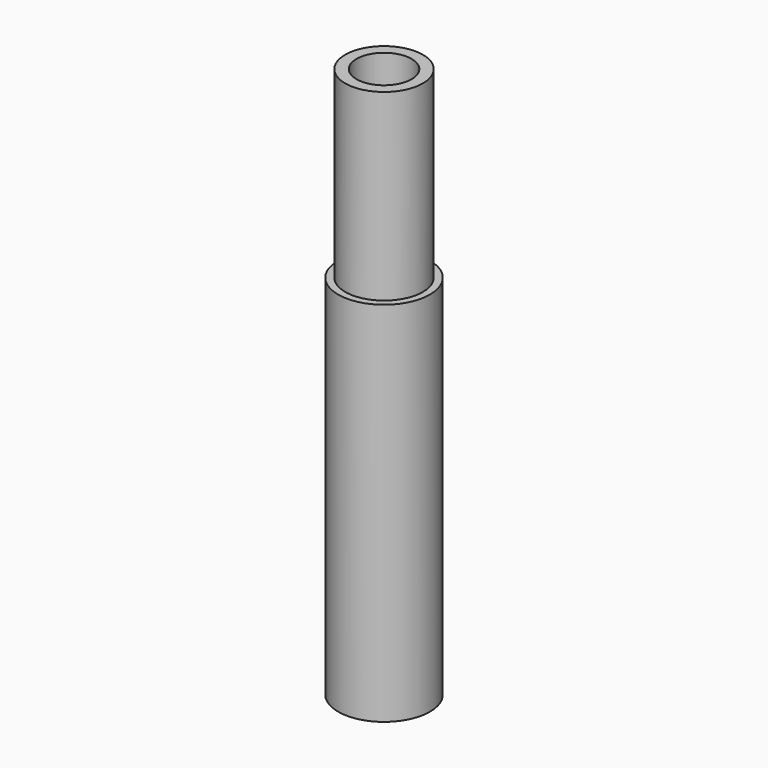
from build123d import *

# Parameters (mm, degrees)
F0_R     = 6.35
F1_DEPTH = 76.2
F2_T     = -2.54
F5_R     = 6.35
F5_R_2   = 5.3717360651
F6_DEPTH = 25.4


# Not quite as in the source:
# - the program builds the solid bodies; features that only make, move or delete a surface that nothing else refers to are left out


with BuildPart() as f1:
    # F0 (on Top) → F1 (new body)
    with BuildSketch(Plane.XY):
        Circle(F0_R)
    extrude(amount=F1_DEPTH)

    # F2
    f2_openings = [f1.faces().sort_by_distance(p)[0] for p in [
        (0, 0, 76.2),
    ]]
    offset(amount=F2_T, openings=f2_openings)

    # F5 (on face) → F6 (cut)
    with BuildSketch(Plane.XY.offset(76.2)):
        Circle(F5_R)
        Circle(F5_R_2, mode=Mode.SUBTRACT)
    extrude(amount=-F6_DEPTH, mode=Mode.SUBTRACT)


solid = f1.part
